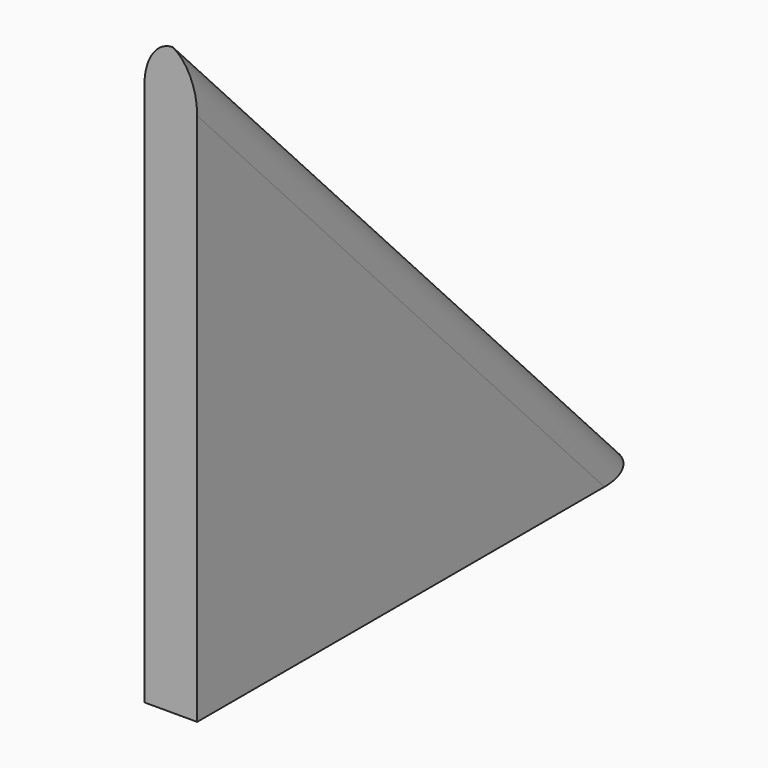
from build123d import *

# Parameters (mm, degrees)
F1_DEPTH    = 4.064
F2_DEPTH    = 2.794
F3_R        = 3.6792614691
F4_T1_DEPTH = 129.0096523961


# Not quite as in the source:
# - a fillet or chamfer that OpenCascade refuses, or shapes differently, is made with other operations: its cross-section is extruded or revolved along the edge and cut away or added


with BuildPart() as f1:
    # F0 (on Right) → F1 (new body)
    with BuildSketch(Plane.YZ):
        Polygon((72.7801844478, 0), (0, 76.3147622347), (0, 0), align=None)
    extrude(amount=F1_DEPTH)

    # F2 (add): a face of the model
    f2_faces = [f1.faces().sort_by_distance(p)[0] for p in [
        (0, 24.2600614826, 25.4382540782),
    ]]
    extrude(f2_faces, amount=F2_DEPTH)

    # F3
    f3_edges = [f1.edges().sort_by_distance(p)[0] for p in [
        (-2.794, 36.390092, 38.157381),
    ]]
    fillet(f3_edges, radius=F3_R)

    # F4: fillet of radius 5.08 on 1 edges, made by hand

    # F4_s2 → F4_t1 (cut)
    with BuildSketch(Plane(origin=(0, 42.7935550314, -44.8718288113), x_dir=(1, 0, 0), z_dir=(0, -0.6901495666, 0.7236667574))):
        with BuildLine():
            ThreePointArc((0.8852614691, 52.6686000807), (3.1949861234, 50.7992812188), (4.064, 47.9578034574))
            Line((4.064, 47.9578034574), (4.064, 52.6686000807))
            Line((4.064, 52.6686000807), (0.8852614691, 52.6686000807))
        make_face()
    extrude(amount=F4_T1_DEPTH, mode=Mode.SUBTRACT)


solid = f1.part
